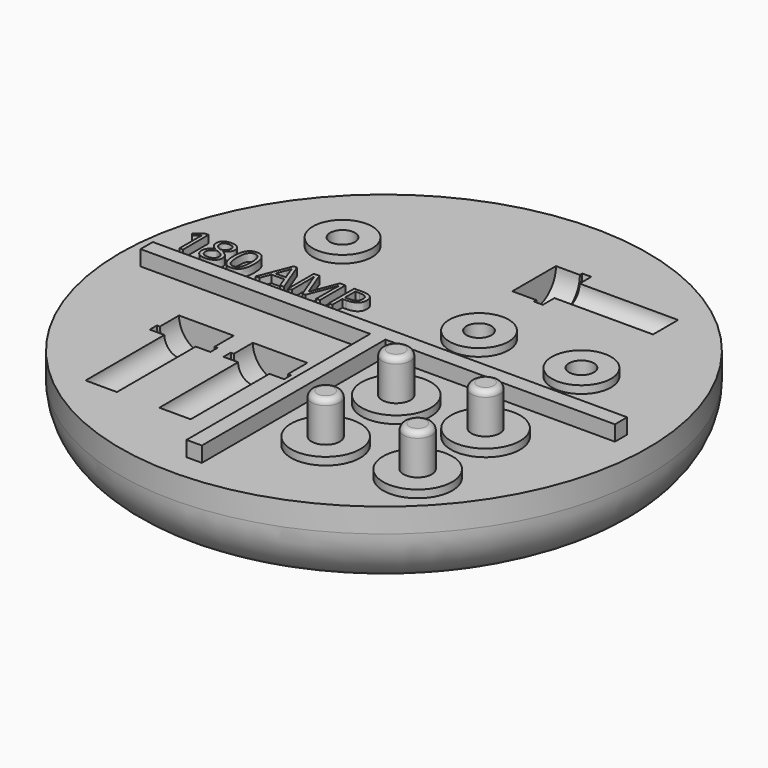
from build123d import *

# Parameters (mm, degrees)
F0_W         = 43
F0_H         = 2
F2_R         = 43
F3_DEPTH     = 2
F4_W         = 4
F4_H         = 2.0122560501
F4_H_2       = 59.9877439499
F5_DEPTH     = 4
F6_TEXT_SIZE = 11.6792921391
F7_DEPTH     = 2
F9_R         = 7.75
F10_DEPTH    = 2
F8_R         = 7.75
F11_DEPTH    = 2
F12_R        = 3.25
F13_DEPTH    = 23.301
F14_R        = 7.75
F15_DEPTH    = 2
F16_R        = 3.25
F17_DEPTH    = 23.301
F18_R        = 7.75
F19_DEPTH    = 2
F20_R        = 3.25
F21_DEPTH    = 23.301
F28_R        = 9.05
F32_DEPTH    = 2
F29_R        = 9.05
F30_R        = 9.05
F33_DEPTH    = 2
F31_R        = 9.05
F34_DEPTH    = 2
F38_R        = 3.7
F39_DEPTH    = 10.5
F35_R        = 3.7
F36_R        = 3.7
F37_R        = 3.7
F40_DEPTH    = 10.5
F41_R        = 1.5


# Not quite as in the source:
# - Text() gives the source's letters only with a copy of the font that has no kerning and outlines rounded to 1/6400 em; it was checked with that copy


with BuildPart() as f1:
    # F0 (on Front) → F1 (revolve)
    with BuildSketch(Plane.XZ):
        with BuildLine():
            Line((0, -19.3), (0, 0))
            Line((0, 0), (-69, 0))
            Line((-69, 0), (-69, -6.3))
            ThreePointArc((-69, -6.3), (-64.6066017178, -16.9066017178), (-54, -21.3))
            Line((-54, -21.3), (-43, -21.3))
            Line((-43, -21.3), (-43, -19.3))
            Line((-43, -19.3), (0, -19.3))
        make_face()
        with Locations((-21.5, -20.3)):
            Rectangle(F0_W, F0_H)
    revolve(axis=Axis((0, 0, -20.3), (0, 0, 1)))

    # F2 (on face) → F3 (cut)
    with BuildSketch(Plane(origin=(0, 0, -21.3), x_dir=(1, 0, 0), z_dir=(0, 0, -1))):
        Circle(F2_R)
    extrude(amount=-F3_DEPTH, mode=Mode.SUBTRACT)

    # F4 (on face) → F5 (join)
    with BuildSketch(Plane.XY):
        Polygon((-2, -2), (-2, 0.0122560501), (2, 0.0122560501), (2, -2), (61.9877439499, -2), (61.9877439499, 2), (-62.02, 2), (-62.02, -2), align=None)
        with Locations((0, -0.993871975)):
            Rectangle(F4_W, F4_H)
        with Locations((0, -31.993871975)):
            Rectangle(F4_W, F4_H_2)
    extrude(amount=F5_DEPTH)

    # F6 (on face) → F7 (join)
    with BuildSketch(Plane.XY):
        with Locations((-61.5909136832, 6.2500005588)):
            Text('180 AMP', F6_TEXT_SIZE, font='Open Sans', text_align=(TextAlign.LEFT, TextAlign.BOTTOM))
    extrude(amount=F7_DEPTH)

    # F9 (on face) → F10 (join)
    with BuildSketch(Plane.XY):
        with Locations((-35.4545451701, 30.7954549789)):
            Circle(F9_R)
    extrude(amount=F10_DEPTH)

    # F8 (on face) → F11 (join)
    with BuildSketch(Plane.XY):
        with Locations((-35.4545451701, 30.7954549789)):
            Circle(F8_R)
    extrude(amount=F11_DEPTH)

    # F12 (on face) → F13 (cut, through all)
    with BuildSketch(Plane.XY.offset(2)):
        with Locations((-35.4545451701, 30.7954549789)):
            Circle(F12_R)
    extrude(amount=-F13_DEPTH, mode=Mode.SUBTRACT)

    # F14 (on face) → F15 (join)
    with BuildSketch(Plane.XY):
        with Locations((12.0454542339, 16.0227268934)):
            Circle(F14_R)
    extrude(amount=F15_DEPTH)

    # F16 (on face) → F17 (cut, through all)
    with BuildSketch(Plane.XY.offset(2)):
        with Locations((12.0454542339, 16.0227268934)):
            Circle(F16_R)
    extrude(amount=-F17_DEPTH, mode=Mode.SUBTRACT)

    # F18 (on face) → F19 (join)
    with BuildSketch(Plane.XY):
        with Locations((38.636367768, 16.2500012666)):
            Circle(F18_R)
    extrude(amount=F19_DEPTH)

    # F20 (on face) → F21 (cut, through all)
    with BuildSketch(Plane.XY.offset(2)):
        with Locations((38.636367768, 16.2500012666)):
            Circle(F20_R)
    extrude(amount=-F21_DEPTH, mode=Mode.SUBTRACT)

    # F22 (on face) → F23 (revolve, cut)
    with BuildSketch(Plane.XY):
        Polygon((10.3409079835, 43.9772754908), (4.0909079835, 43.9772754908), (4.0909079835, 36.8522754908), (10.3409079835, 36.8522754908), (10.3409079835, 36.0522754908), (12.6909079835, 36.0522754908), (12.6909079835, 39.8772754908), (38.4409079835, 39.8772754908), (38.4409079835, 43.9772754908), (12.6909079835, 43.9772754908), align=None)
    revolve(axis=Axis((25.5659079835, 43.9772754908, 0), (1, 0, 0)), mode=Mode.SUBTRACT)

    # F24 (on face) → F25 (revolve, cut)
    with BuildSketch(Plane.XY):
        Polygon((-15.925, -22.6136371493), (-15.925, -48.3636371493), (-11.825, -48.3636371493), (-11.825, -22.6136371493), (-8, -22.6136371493), (-8, -20.2636371493), (-8.8, -20.2636371493), (-8.8, -14.0136371493), (-15.925, -14.0136371493), (-15.925, -20.2636371493), align=None)
    revolve(axis=Axis((-15.925, -35.4886371493, 0), (0, -1, 0)), mode=Mode.SUBTRACT)

    # F26 (on face) → F27 (revolve, cut)
    with BuildSketch(Plane.XY):
        Polygon((-28.05, -14.0136371493), (-35.2, -14.0136371493), (-35.2, -20.2636371493), (-35.2, -22.6136371493), (-35.2, -48.3636371493), (-31.1, -48.3636371493), (-31.1, -22.6136371493), (-27.275, -22.6136371493), (-27.275, -20.2636371493), (-28.05, -20.2636371493), align=None)
    revolve(axis=Axis((-35.2, -35.4886371493, 0), (0, -1, 0)), mode=Mode.SUBTRACT)

    # F28 (on face) → F32 (join)
    with BuildSketch(Plane.XY):
        with Locations((16.6225461161, -16.7441392301)):
            Circle(F28_R)
    extrude(amount=F32_DEPTH)

    # F29 (on face) + F30 (on face) → F33 (join)
    with BuildSketch(Plane.XY):
        with Locations((40.0214559379, -16.8149948486)):
            Circle(F29_R)
    with BuildSketch(Plane.XY):
        with Locations((16.8163470961, -40.0522500635)):
            Circle(F30_R)
    extrude(amount=F33_DEPTH)

    # F31 (on face) → F34 (join)
    with BuildSketch(Plane.XY):
        with Locations((40.5137918128, -39.6079486627)):
            Circle(F31_R)
    extrude(amount=F34_DEPTH)

    # F38 (on face) → F39 (join)
    with BuildSketch(Plane.XY.offset(2)):
        with Locations((40.0214559379, -16.8149948486)):
            Circle(F38_R)
    extrude(amount=F39_DEPTH)

    # F35 (on face) + F36 (on face) + F37 (on face) → F40 (join)
    with BuildSketch(Plane.XY.offset(2)):
        with Locations((16.6225461161, -16.7441392301)):
            Circle(F35_R)
    with BuildSketch(Plane.XY.offset(2)):
        with Locations((16.8163470961, -40.0522500635)):
            Circle(F36_R)
    with BuildSketch(Plane.XY.offset(2)):
        with Locations((40.5137918128, -39.6079486627)):
            Circle(F37_R)
    extrude(amount=F40_DEPTH)

    # F41
    f41_edges = [f1.edges().sort_by_distance(p)[0] for p in [
        (13.116347, -40.05225, 12.5),
        (12.922546, -16.744139, 12.5),
        (36.321456, -16.814995, 12.5),
        (36.813792, -39.607949, 12.5),
    ]]
    fillet(f41_edges, radius=F41_R)


solid = f1.part
